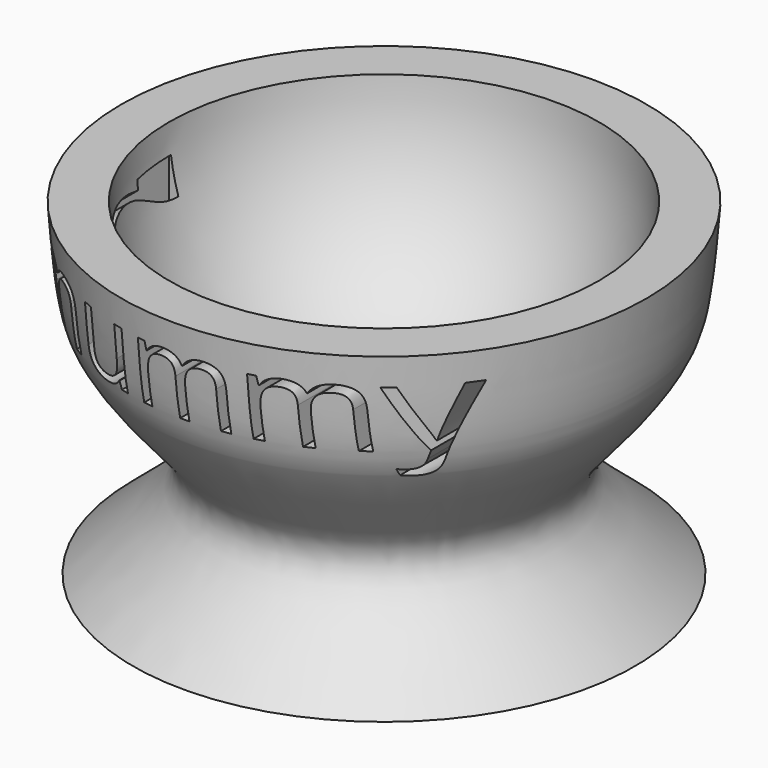
from build123d import *

# Parameters (mm, degrees)
F2_TEXT_SIZE = 11.8327367137
F3_DEPTH     = 50.5


# Not quite as in the source:
# - Text() gives the source's letters only with a copy of the font that has no kerning and outlines rounded to 1/6400 em; it was checked with that copy


with BuildPart() as f1:
    # F0 (on Front) → F1 (revolve)
    with BuildSketch(Plane.XZ):
        with BuildLine():
            Line((-26.2838205291, 0), (0, 0))
            Line((0, 0), (0, 11.7869073588))
            ThreePointArc((0, 11.7869073588), (-15.9099025767, 18.3770047821), (-22.5, 34.2869073588))
            Line((-22.5, 34.2869073588), (-27.5, 34.2869073588))
            add(Edge.make_bspline(
                [(-27.5, 34.2869073588), (-26.8992389282, 26.4769974726), (-26.4909277035, 22.8004791877), (-20.2764636175, 15.1729285166), (-17.2940219488, 12.0217100187), (-16.9237361055, 7.4337774517), (-23.4051413829, 2.4788607444), (-26.2838205291, 0)],
                knots=[0, 0, 0, 0, 0.258330667, 0.4658353106, 0.6147523547, 0.7522245371, 1, 1, 1, 1], degree=3))
        make_face()
    revolve(axis=Axis((0, 0, 17.1434536794), (0, 0, 1)))

    # F2 (on Front) → F3 (cut)
    with BuildSketch(Plane.XZ):
        with Locations((-23.5, 25)):
            Text('mummy', F2_TEXT_SIZE, font='Open Sans', text_align=(TextAlign.LEFT, TextAlign.BOTTOM))
    extrude(amount=F3_DEPTH, mode=Mode.SUBTRACT)


solid = f1.part
